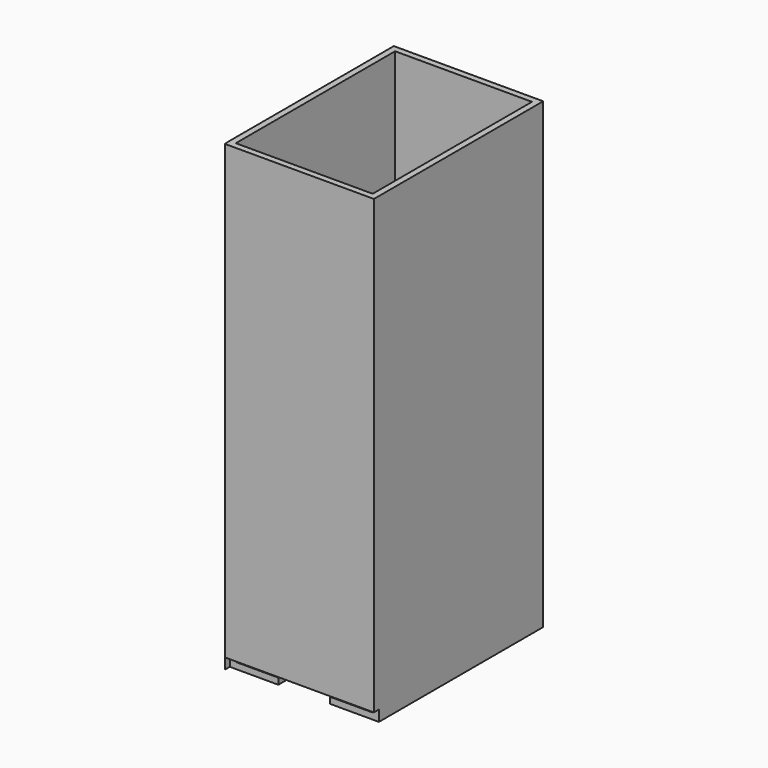
from build123d import *

# Parameters (mm, degrees)
F0_W     = 3.175
F0_H     = 101.6
F1_DEPTH = 228.6
F2_DEPTH = 236.22
F0_W_2   = 21.717
F3_DEPTH = 3.175
F4_W     = 76.0733831866
F4_H     = 5.55625
F5_DEPTH = 3.175


# Not quite as in the source:
# - the program builds the solid bodies; features that only make, move or delete a surface that nothing else refers to are left out


with BuildPart() as f1:
    # F0 (on Top) → F1 (new body)
    with BuildSketch(Plane.XY):
        with Locations((36.5125, -2.4078887083)):
            Rectangle(F0_W, F0_H)
    extrude(amount=F1_DEPTH)

    # F0 (on Top) → F2 (join)
    with BuildSketch(Plane.XY):
        Polygon((-34.925, 48.3921112917), (-13.208, 48.3921112917), (13.208, 48.3921112917), (34.925, 48.3921112917), (38.1, 48.3921112917), (38.1, 51.5671112917), (-38.1, 51.5671112917), (-38.1, 48.3921112917), align=None)
        Polygon((-34.925, -53.2078887083), (-34.925, 48.3921112917), (-38.1, 48.3921112917), (-38.1, -53.3400028944), align=None)
        Polygon((13.208, -53.2078887083), (-13.208, -53.2078887083), (-34.925, -53.2078887083), (-38.1, -53.3400028944), (-37.9733831866, -56.3828887083), (38.1, -56.3828887083), (38.1, -53.2078887083), (34.925, -53.2078887083), align=None)
        with Locations((36.5125, -2.4078887083)):
            Rectangle(F0_W, F0_H)
    extrude(amount=F2_DEPTH)

    # F0 (on Top) → F3 (join)
    with BuildSketch(Plane.XY):
        with Locations((-24.0665, -2.4078887083)):
            Rectangle(F0_W_2, F0_H)
        with Locations((24.0665, -2.4078887083)):
            Rectangle(F0_W_2, F0_H)
    extrude(amount=F3_DEPTH)

    # F4 (on face) → F5 (cut)
    with BuildSketch(Plane.XZ.offset(56.3828887083)):
        with Locations((0.0633084067, 2.778125)):
            Rectangle(F4_W, F4_H)
    extrude(amount=-F5_DEPTH, mode=Mode.SUBTRACT)


solid = f1.part
